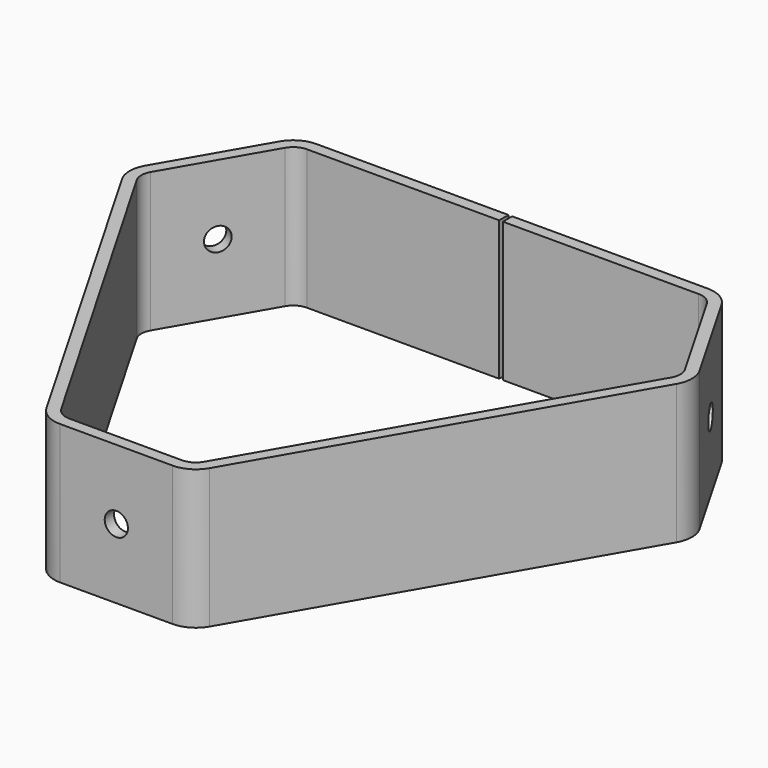
from build123d import *

# Parameters (mm, degrees)
F1_W     = 1
F1_H     = 12
F3_R     = 1
F4_DEPTH = 1
F5_R     = 1
F6_DEPTH = 1
F7_R     = 1
F8_DEPTH = 1


with BuildPart() as f2:
    # F2: sweep along a path in F0
    with BuildLine(Plane.XY) as f2_path:
        Line((0, 17.3205080757), (0.268994947, 17.3205080757))
        Line((0.268994947, 17.3205080757), (16.8452994616, 17.3205080757))
        ThreePointArc((16.8452994616, 17.3205080757), (17.8461933486, 17.0520424897), (18.5783816717, 16.3187195027))
        Line((18.5783816717, 16.3187195027), (23.4179019593, 7.9164048343))
        ThreePointArc((23.4179019593, 7.9164048343), (23.6848194828, 6.9171610817), (23.4168705568, 5.9181934072))
        Line((23.4168705568, 5.9181934072), (6.5773502692, -23.248711306))
        ThreePointArc((6.5773502692, -23.248711306), (5.8452994616, -23.9807621135), (4.8452994616, -24.248711306))
        Line((4.8452994616, -24.248711306), (-4.8452994616, -24.248711306))
        ThreePointArc((-4.8452994616, -24.248711306), (-5.8452994616, -23.9807621135), (-6.5773502692, -23.248711306))
        Line((-6.5773502692, -23.248711306), (-23.4226497308, 5.9282032303))
        ThreePointArc((-23.4226497308, 5.9282032303), (-23.6905989232, 6.9282032303), (-23.4226497308, 7.9282032303))
        Line((-23.4226497308, 7.9282032303), (-18.5773502692, 16.3205080757))
        ThreePointArc((-18.5773502692, 16.3205080757), (-17.8452994616, 17.0525588833), (-16.8452994616, 17.3205080757))
        Line((-16.8452994616, 17.3205080757), (-0.3151426208, 17.3205080757))
    # F1 (on Right) → F2 (sweep)
    with BuildSketch(Plane.YZ):
        with Locations((17.3205080757, 0)):
            Rectangle(F1_W, F1_H)
    sweep(path=f2_path.line)

    # F3 (on face) → F4 (cut, through all)
    with BuildSketch(Plane.XZ.offset(24.748711306)):
        Circle(F3_R)
    extrude(amount=-F4_DEPTH, mode=Mode.SUBTRACT)

    # F5 (on face) → F6 (cut, through all)
    with BuildSketch(Plane(origin=(21.441430996, 12.3497208085, 0), x_dir=(-0.4991057135, 0.866541105, 0), z_dir=(0.866541105, 0.4991057135, 0))):
        Circle(F5_R)
    extrude(amount=-F6_DEPTH, mode=Mode.SUBTRACT)

    # F7 (on face) → F8 (cut, through all)
    with BuildSketch(Plane(origin=(-21.4330127019, 12.374355653, 0), x_dir=(-0.5, -0.8660254038, 0), z_dir=(-0.8660254038, 0.5, 0))):
        Circle(F7_R)
    extrude(amount=-F8_DEPTH, mode=Mode.SUBTRACT)


solid = f2.part
